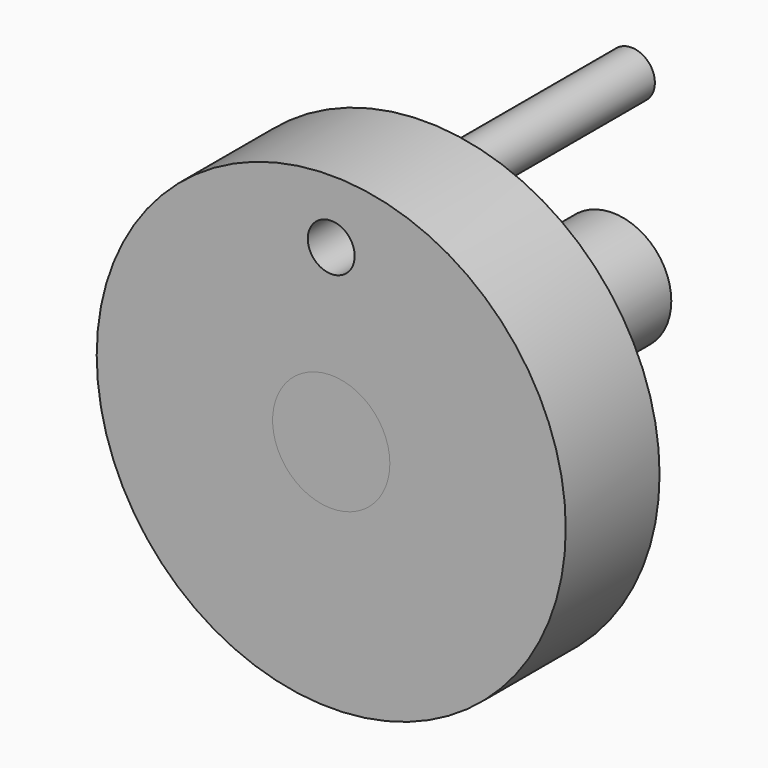
from build123d import *

# Parameters (mm, degrees)
F0_R     = 25.4
F0_R_2   = 6.35
F0_R_3   = 2.54
F1_DEPTH = 12.7
F2_R     = 6.35
F3_DEPTH = 38.1
F5_R     = 2.54
F6_DEPTH = 27.94


with BuildPart() as f1:
    # F0 (on Front) → F1 (new body)
    with BuildSketch(Plane.XZ):
        Circle(F0_R)
        Circle(F0_R_2, mode=Mode.SUBTRACT)
        with Locations((0, 18.5419153422)):
            Circle(F0_R_3, mode=Mode.SUBTRACT)
    extrude(amount=F1_DEPTH)


with BuildPart() as f3:
    # F2 (on face) → F3 (new body)
    with BuildSketch(Plane.XZ.offset(12.7)):
        Circle(F2_R)
    extrude(amount=-F3_DEPTH)


with BuildPart() as f6:
    # F5 (on face) → F6 (new body)
    with BuildSketch(Plane(origin=(0, 0, 0), x_dir=(-1, 0, 0), z_dir=(0, 1, 0))):
        with Locations((0, 18.5419153422)):
            Circle(F5_R)
    extrude(amount=F6_DEPTH)


solid = Compound([f1.part, f3.part, f6.part])
